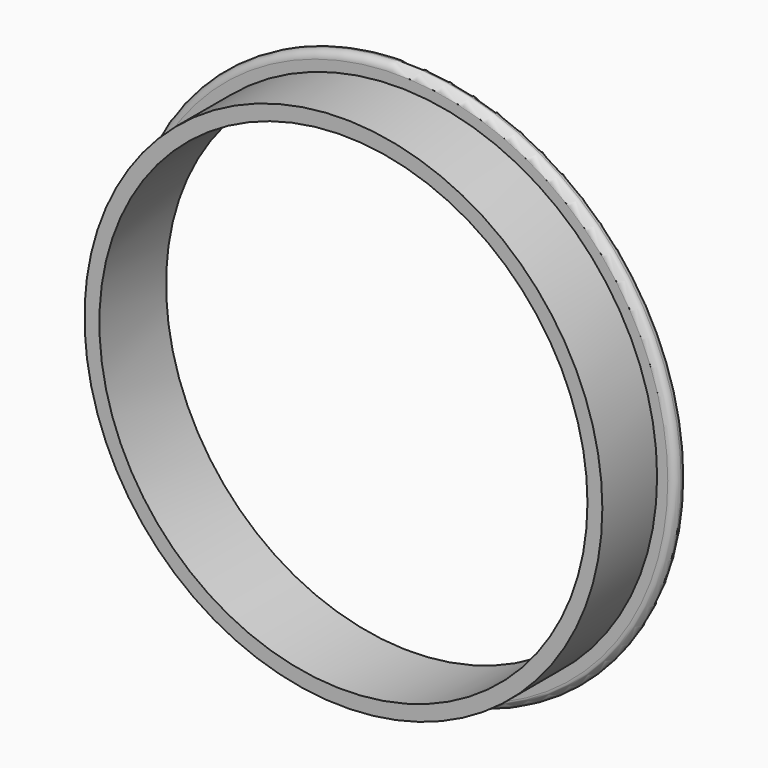
from build123d import *

# Parameters (mm, degrees)
F0_R     = 43.5
F0_R_2   = 41
F1_DEPTH = 14
F0_R_3   = 46.5412209473
F2_DEPTH = 2.5
F3_R     = 1.24999


# Not quite as in the source:
# - a fillet or chamfer is up to 0.001 mm smaller than in the source, because OpenCascade refuses the exact size


with BuildPart() as f1:
    # F0 (on Front) → F1 (new body)
    with BuildSketch(Plane.XZ):
        Circle(F0_R)
        Circle(F0_R_2, mode=Mode.SUBTRACT)
    extrude(amount=F1_DEPTH)

    # F0 (on Front) → F2 (join)
    with BuildSketch(Plane.XZ):
        Circle(F0_R_3)
        Circle(F0_R, mode=Mode.SUBTRACT)
    extrude(amount=F2_DEPTH)

    # F3 (radius 1.25 in the source; OpenCascade refuses exactly that, so slightly less here)
    f3_edges = [f1.edges().sort_by_distance(p)[0] for p in [
        (-46.541221, -2.5, 0),
        (-46.541221, 0, 0),
    ]]
    fillet(f3_edges, radius=F3_R)


solid = f1.part
